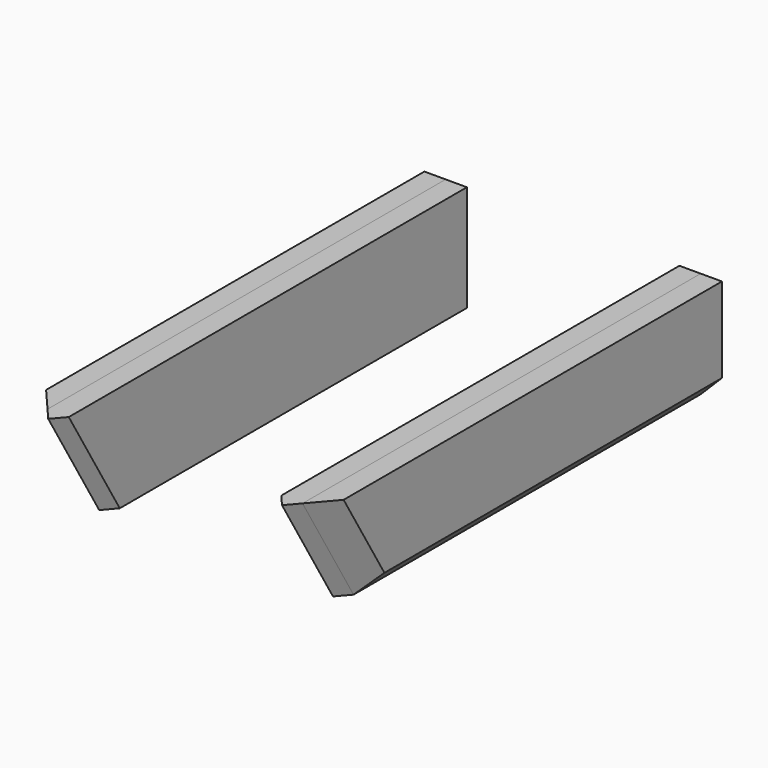
from build123d import *

# Parameters (mm, degrees)
F1_DEPTH = 12.7
F2_SIZE2 = 6.35
F2_SIZE  = 6.35
F3_SIZE2 = 6.34999
F3_SIZE  = 6.34999
F5_DEPTH = 12.7
F6_SIZE2 = 12.69999
F6_SIZE  = 12.69999
F7_SIZE2 = 12.69999
F7_SIZE  = 12.69999


# Not quite as in the source:
# - a fillet or chamfer is up to 0.001 mm smaller than in the source, because OpenCascade refuses the exact size


with BuildPart() as f1:
    # F0 (on Right) → F1 (new body)
    with BuildSketch(Plane.YZ):
        Polygon((152.4, 31.75), (-152.4, 31.75), (-114.3, -31.75), (152.4, -31.75), align=None)
    extrude(amount=F1_DEPTH)

    # F2
    f2_edges = [f1.edges().sort_by_distance(p)[0] for p in [
        (12.7, -133.35, 0),
    ]]
    chamfer(f2_edges, length=F2_SIZE, length2=F2_SIZE2)

    # F3 (size 6.35 and 6.35 in the source; OpenCascade refuses exactly that, so slightly less here)
    f3_edges = [f1.edges().sort_by_distance(p)[0] for p in [
        (0, -133.35, 0),
    ]]
    chamfer(f3_edges, length=F3_SIZE, length2=F3_SIZE2)


with BuildPart() as f5:
    # F4 (on face) → F5 (new body)
    with BuildSketch(Plane.YZ.offset(12.7)):
        Polygon((152.4, 31.75), (-144.9946910935, 31.75), (-106.8946910935, -31.75), (152.4, -31.75), align=None)
    extrude(amount=F5_DEPTH)

    # F6 (size 12.7 and 12.7 in the source; OpenCascade refuses exactly that, so slightly less here)
    f6_edges = [f5.edges().sort_by_distance(p)[0] for p in [
        (25.4, -125.944691, 0),
    ]]
    chamfer(f6_edges, length=F6_SIZE, length2=F6_SIZE2)

    # F7 (size 12.7 and 12.7 in the source; OpenCascade refuses exactly that, so slightly less here)
    f7_edges = [f5.edges().sort_by_distance(p)[0] for p in [
        (25.4, 30.157958, -31.75),
    ]]
    chamfer(f7_edges, length=F7_SIZE, length2=F7_SIZE2)


with BuildPart() as f1_1:
    # F8: moved
    add(f1.part.moved(Location((63.5, 0, 0))))


with BuildPart() as f5_1:
    # F8: moved
    add(f5.part.moved(Location((63.5, 0, 0))))


with BuildPart() as f9_1:
    # F9: instance of F1
    add(f1_1.part.mirror(Plane.YZ))


with BuildPart() as f9_2:
    # F9: instance of F5
    add(f5_1.part.mirror(Plane.YZ))


solid = Compound([f1_1.part, f5_1.part, f9_1.part, f9_2.part])
